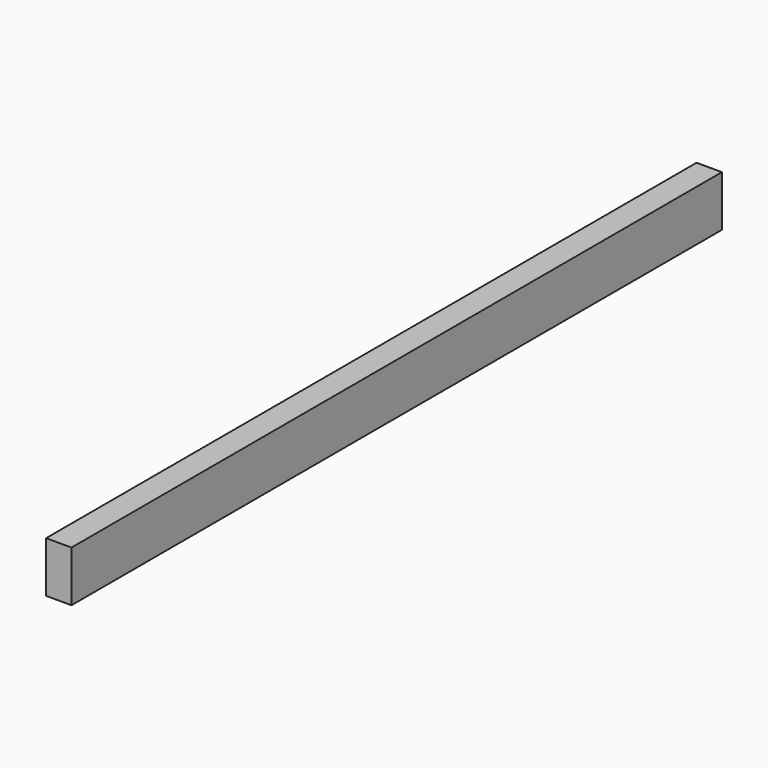
from build123d import *

# Parameters (mm, degrees)
F1_W     = 19.05
F1_H     = 38.1
F2_DEPTH = 609.6


# Not quite as in the source:
# - a variable given as a bare number and used for a length is read in inches; the dataset says mm whatever the document's units were


with BuildPart() as f2:
    # F1 (on Front) → F2 (new body)
    with BuildSketch(Plane.XZ):
        with Locations((9.525, 19.05)):
            Rectangle(F1_W, F1_H)
    extrude(amount=F2_DEPTH)


solid = f2.part
